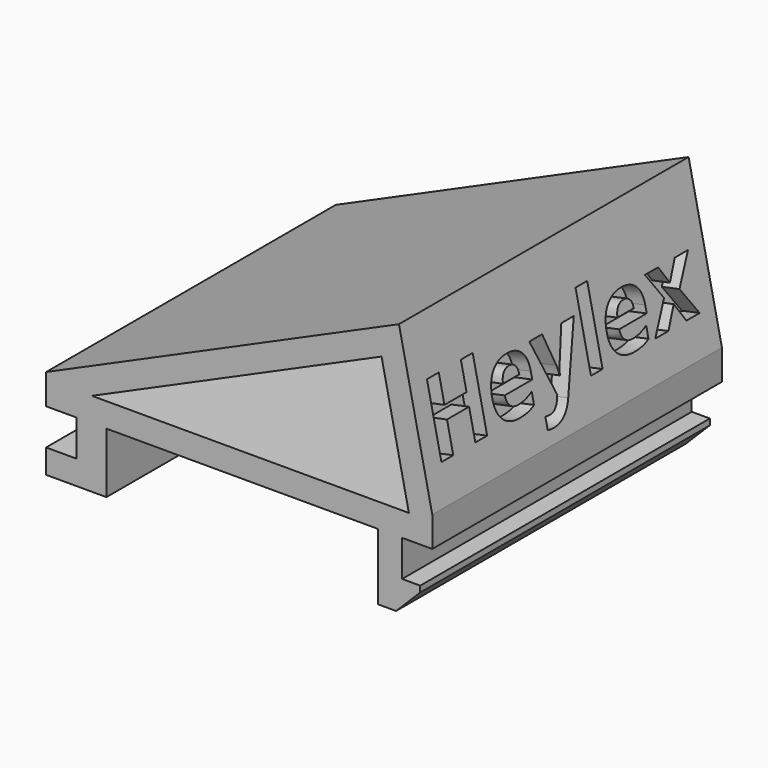
from build123d import *

# Parameters (mm, degrees)
F1_DEPTH     = 30
F2_SIZE      = 2
F3_TEXT_SIZE = 8.0950444956
F4_DEPTH     = 1.5


# Not quite as in the source:
# - Text() gives the source's letters only with a copy of the font that has no kerning and outlines rounded to 1/6400 em; it was checked with that copy


with BuildPart() as f1:
    # F0 (on Front) → F1 (new body)
    with BuildSketch(Plane.XZ):
        Polygon((-16.0259055989, 2.5), (-16.0259055989, 0), (-13.5259055989, 0), (-13.5259055989, -3), (-16.0259055989, -3), (-16.0259055989, -5), (-11.0259055989, -5), (-11.0259055989, 0), (11.4715139763, 0), (11.4715139763, -5.5), (14.9740944011, -5.5), (14.9740944011, -3), (13.4740944011, -3), (13.4740944011, 0), (15.9740944011, 0), (15.9740944011, 2.5), (13.2144774356, 15.5), align=None)
        Polygon((13.9715138066, 2), (-12.2274587925, 2), (11.7707876706, 12.6693952556), (14.0356679906, 2), align=None, mode=Mode.SUBTRACT)
    extrude(amount=F1_DEPTH)

    # F2
    f2_edges = [f1.edges().sort_by_distance(p)[0] for p in [
        (14.974094, -15, -5.5),
    ]]
    chamfer(f2_edges, length=F2_SIZE)

    # F3 (on face) → F4 (cut)
    with BuildSketch(Plane(origin=(15.7931196837, 0, 3.352535463), x_dir=(0, 1, 0), z_dir=(0.9782029365, 0, 0.2076511861))):
        with Locations((-29, 2.128467692)):
            Text('Heylex', F3_TEXT_SIZE, font='Open Sans', font_style=FontStyle.BOLD, text_align=(TextAlign.LEFT, TextAlign.BOTTOM))
    extrude(amount=-F4_DEPTH, mode=Mode.SUBTRACT)


solid = f1.part
